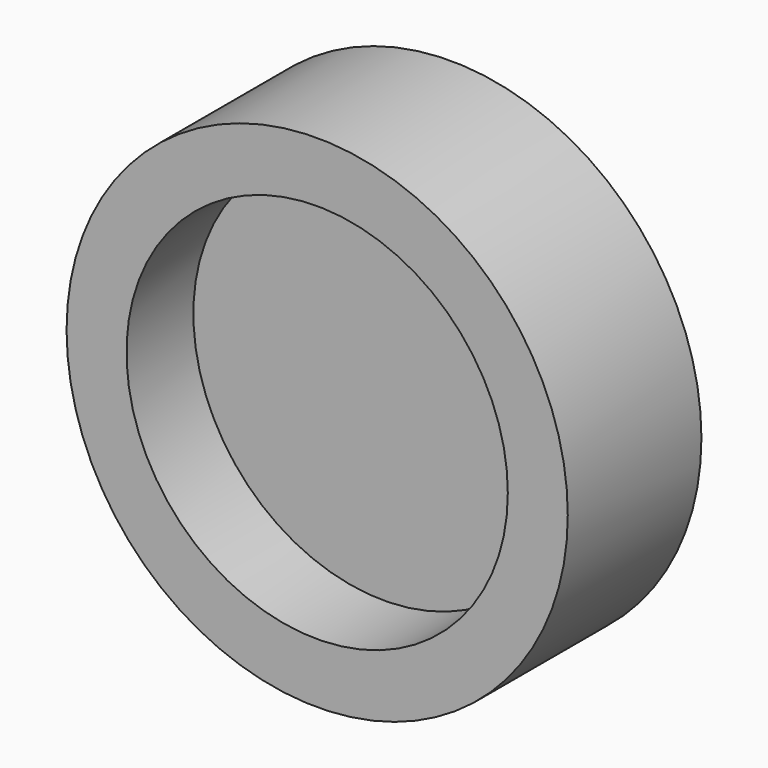
from build123d import *

# Parameters (mm, degrees)
F0_R     = 38.1
F1_DEPTH = 25.4
F2_R     = 28.9854194273
F3_DEPTH = 12.7


# Not quite as in the source:
# - the program builds the solid bodies; features that only make, move or delete a surface that nothing else refers to are left out


with BuildPart() as f1:
    # F0 (on Front) → F1 (new body)
    with BuildSketch(Plane.XZ):
        Circle(F0_R)
    extrude(amount=F1_DEPTH)

    # F2 (on face) → F3 (cut)
    with BuildSketch(Plane.XZ.offset(25.4)):
        Circle(F2_R)
    extrude(amount=-F3_DEPTH, mode=Mode.SUBTRACT)


solid = f1.part
